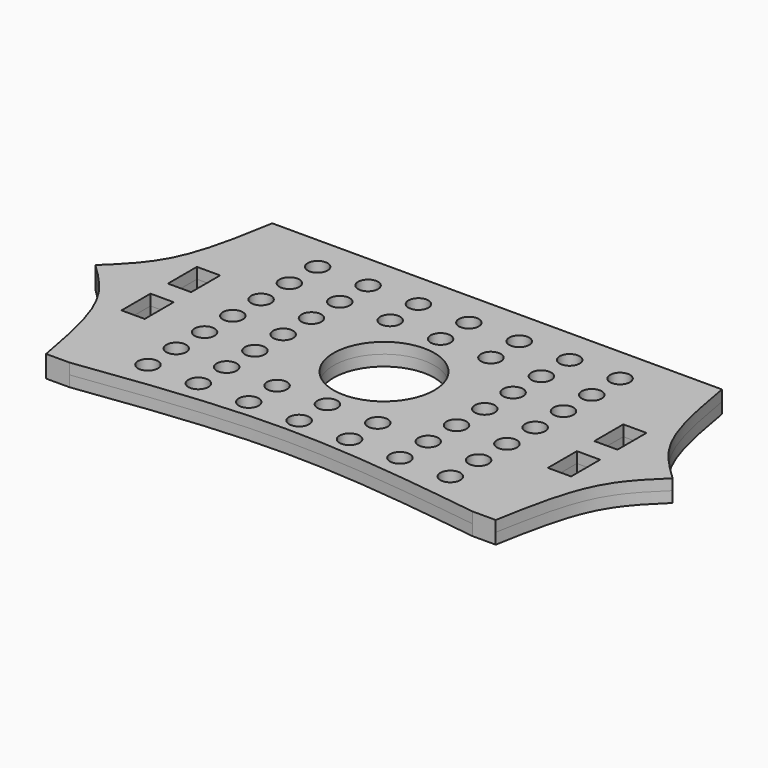
from build123d import *

# Parameters (mm, degrees)
F0_R     = 1.375
F0_R_2   = 6.95
F1_DEPTH = 1.5


with BuildPart() as f1:
    # F0 (on Top) → F1 (new body, symmetric)
    with BuildSketch(Plane.XY):
        with BuildLine():
            Line((-31, -19.5), (-27.8, -19.5))
            add(Edge.make_bspline(
                [(-27.8, -19.5), (-18.5333333333, -18.25), (0, -15.75), (18.5333333333, -18.25), (27.8, -19.5)],
                knots=[0, 0, 0, 0, 0.5, 1, 1, 1, 1], degree=3))
            Line((27.8, -19.5), (31, -19.5))
            add(Edge.make_bspline(
                [(39.8, 0), (37.8467765607, -1.8901869566), (33.4188629122, -6.1751983155), (31.8671997538, -14.7228525715), (31, -19.5)],
                knots=[0, 0, 0, 0, 0.4411159734, 1, 1, 1, 1], degree=3))
            add(Edge.make_bspline(
                [(31, 19.5), (31.8282806058, 14.7207922386), (33.3126793566, 6.1557600729), (37.8114855459, 1.8868834383), (39.8, 0)],
                knots=[0, 0, 0, 0, 0.5579906379, 1, 1, 1, 1], degree=3))
            Line((31, 19.5), (27.8, 19.5))
            Line((27.8, 19.5), (-27.8, 19.5))
            Line((-27.8, 19.5), (-31, 19.5))
            add(Edge.make_bspline(
                [(-31, 19.5), (-31.8282806058, 14.7207922386), (-33.3126793566, 6.1557600729), (-37.8114855459, 1.8868834383), (-39.8, 0)],
                knots=[0, 0, 0, 0, 0.5579906379, 1, 1, 1, 1], degree=3))
            add(Edge.make_bspline(
                [(-31, -19.5), (-31.8671997538, -14.7228525715), (-33.4188629122, -6.1751983155), (-37.8467765607, -1.8901869566), (-39.8, 0)],
                knots=[0, 0, 0, 0, 0.5588840266, 1, 1, 1, 1], degree=3))
        make_face()
        with Locations((-20.85, -14.625)):
            Circle(F0_R, mode=Mode.SUBTRACT)
        with Locations((-13.9, -14.625)):
            Circle(F0_R, mode=Mode.SUBTRACT)
        with Locations((-6.95, -14.625)):
            Circle(F0_R, mode=Mode.SUBTRACT)
        with Locations((-20.85, -9.75)):
            Circle(F0_R, mode=Mode.SUBTRACT)
        Polygon((-27.8, -3.3), (-27.8, -6.5), (-31, -6.5), (-31, -3.3), (-31, -1.5), (-27.8, -1.5), align=None, mode=Mode.SUBTRACT)
        with Locations((-20.85, -4.875)):
            Circle(F0_R, mode=Mode.SUBTRACT)
        with Locations((-13.9, -9.75)):
            Circle(F0_R, mode=Mode.SUBTRACT)
        with Locations((-6.95, -9.75)):
            Circle(F0_R, mode=Mode.SUBTRACT)
        with Locations((-13.9, -4.875)):
            Circle(F0_R, mode=Mode.SUBTRACT)
        with Locations((0, -14.625)):
            Circle(F0_R, mode=Mode.SUBTRACT)
        with Locations((6.95, -14.625)):
            Circle(F0_R, mode=Mode.SUBTRACT)
        with Locations((13.9, -14.625)):
            Circle(F0_R, mode=Mode.SUBTRACT)
        with Locations((20.85, -14.625)):
            Circle(F0_R, mode=Mode.SUBTRACT)
        with Locations((0, -9.75)):
            Circle(F0_R, mode=Mode.SUBTRACT)
        with Locations((6.95, -9.75)):
            Circle(F0_R, mode=Mode.SUBTRACT)
        with Locations((13.9, -9.75)):
            Circle(F0_R, mode=Mode.SUBTRACT)
        with Locations((13.9, -4.875)):
            Circle(F0_R, mode=Mode.SUBTRACT)
        with Locations((20.85, -9.75)):
            Circle(F0_R, mode=Mode.SUBTRACT)
        with Locations((20.85, -4.875)):
            Circle(F0_R, mode=Mode.SUBTRACT)
        Polygon((31, -3.3), (31, -6.5), (27.8, -6.5), (27.8, -4.875), (27.8, -3.3), (27.8, -1.5), (31, -1.5), align=None, mode=Mode.SUBTRACT)
        with Locations((-20.85, 0)):
            Circle(F0_R, mode=Mode.SUBTRACT)
        Polygon((-27.8, 1.8441202119), (-27.8, 1.5), (-31, 1.5), (-31, 3.6441202119), (-31, 6.5), (-27.8, 6.5), (-27.8, 4.875), align=None, mode=Mode.SUBTRACT)
        with Locations((-20.85, 4.875)):
            Circle(F0_R, mode=Mode.SUBTRACT)
        with Locations((-13.9, 0)):
            Circle(F0_R, mode=Mode.SUBTRACT)
        with Locations((-13.9, 4.875)):
            Circle(F0_R, mode=Mode.SUBTRACT)
        with Locations((-20.85, 9.75)):
            Circle(F0_R, mode=Mode.SUBTRACT)
        with Locations((-20.85, 14.625)):
            Circle(F0_R, mode=Mode.SUBTRACT)
        with Locations((-13.9, 9.75)):
            Circle(F0_R, mode=Mode.SUBTRACT)
        with Locations((-6.95, 9.75)):
            Circle(F0_R, mode=Mode.SUBTRACT)
        with Locations((-13.9, 14.625)):
            Circle(F0_R, mode=Mode.SUBTRACT)
        with Locations((-6.95, 14.625)):
            Circle(F0_R, mode=Mode.SUBTRACT)
        Circle(F0_R_2, mode=Mode.SUBTRACT)
        with Locations((13.9, 0)):
            Circle(F0_R, mode=Mode.SUBTRACT)
        with Locations((13.9, 4.875)):
            Circle(F0_R, mode=Mode.SUBTRACT)
        with Locations((20.85, 0)):
            Circle(F0_R, mode=Mode.SUBTRACT)
        Polygon((27.8, 3.3), (27.8, 6.5), (31, 6.5), (31, 1.5), (27.8, 1.5), align=None, mode=Mode.SUBTRACT)
        with Locations((20.85, 4.875)):
            Circle(F0_R, mode=Mode.SUBTRACT)
        with Locations((0, 9.75)):
            Circle(F0_R, mode=Mode.SUBTRACT)
        with Locations((6.95, 9.75)):
            Circle(F0_R, mode=Mode.SUBTRACT)
        with Locations((13.9, 9.75)):
            Circle(F0_R, mode=Mode.SUBTRACT)
        with Locations((0, 14.625)):
            Circle(F0_R, mode=Mode.SUBTRACT)
        with Locations((6.95, 14.625)):
            Circle(F0_R, mode=Mode.SUBTRACT)
        with Locations((13.9, 14.625)):
            Circle(F0_R, mode=Mode.SUBTRACT)
        with Locations((20.85, 9.75)):
            Circle(F0_R, mode=Mode.SUBTRACT)
        with Locations((20.85, 14.625)):
            Circle(F0_R, mode=Mode.SUBTRACT)
    extrude(amount=F1_DEPTH, both=True)


solid = f1.part
